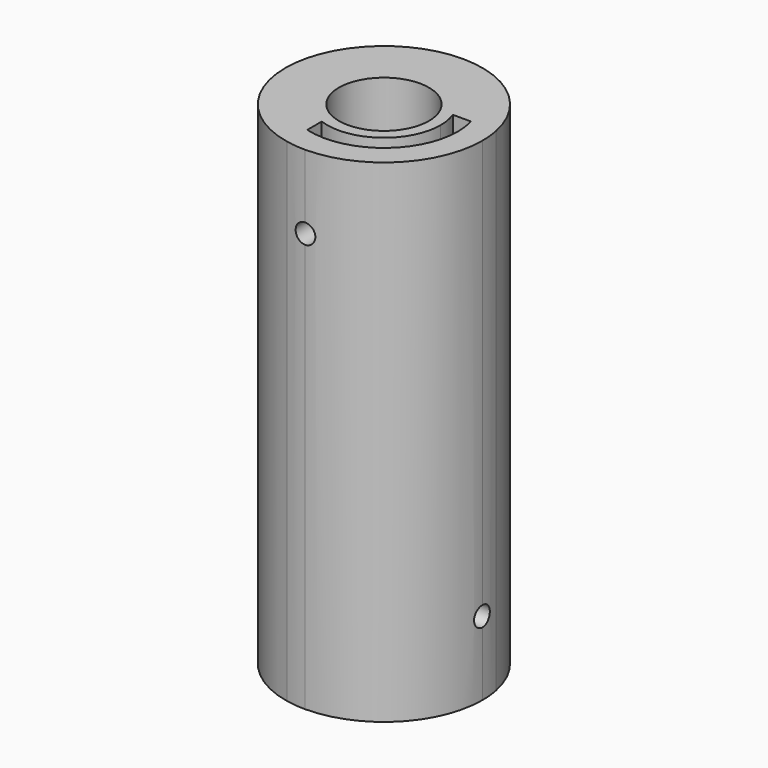
from build123d import *
from build123d import SkipClean  # not in build123d's __all__

# Parameters (mm, degrees)
F1_DEPTH = 100
F2_R     = 2
F3_DEPTH = 15
F4_R     = 2
F5_DEPTH = 6
F6_DEPTH = 100.0010001
F8_R     = 2
F9_DEPTH = 10


with BuildPart() as f1:
    # F0 (on Top) → F1 (new body)
    with BuildSketch(Plane.XY):
        with BuildLine():
            ThreePointArc((-36.113968879, 21.9828632864), (-38.5839959268, 36.6822584753), (-23.884600738, 34.2122314274))
            Line((-23.884600738, 34.2122314274), (-21.3320395526, 34.2122314274))
            ThreePointArc((-21.3320395526, 34.2122314274), (-40.2456968626, 38.3439594111), (-36.113968879, 19.430302101))
            Line((-36.113968879, 19.430302101), (-36.113968879, 21.9828632864))
        make_face()
        with BuildLine():
            ThreePointArc((-23.884600738, 34.2122314274), (-23.1970967118, 32.2645205774), (-22.963968879, 30.2122314274))
            ThreePointArc((-22.963968879, 30.2122314274), (-27.2599756775, 22.4558630762), (-36.113968879, 21.9828632864))
            Line((-36.113968879, 21.9828632864), (-36.113968879, 19.430302101))
            ThreePointArc((-36.113968879, 19.430302101), (-25.5470061107, 20.7716276332), (-20.613968879, 30.2122314274))
            ThreePointArc((-20.613968879, 30.2122314274), (-20.7949100123, 32.2442024836), (-21.3320395526, 34.2122314274))
            Line((-21.3320395526, 34.2122314274), (-23.884600738, 34.2122314274))
        make_face()
        with BuildLine():
            ThreePointArc((-52.113968879, 30.2122314274), (-46.2561045027, 44.3543670512), (-32.113968879, 50.2122314274))
            Line((-32.113968879, 50.2122314274), (-52.113968879, 50.2122314274))
            Line((-52.113968879, 50.2122314274), (-52.113968879, 30.2122314274))
        make_face()
        with BuildLine():
            ThreePointArc((-32.113968879, 50.2122314274), (-19.4648582383, 45.7041648123), (-12.5180509367, 34.2122314274))
            ThreePointArc((-12.5180509367, 34.2122314274), (-12.2152458189, 32.2224106675), (-12.113968879, 30.2122314274))
            Line((-12.113968879, 30.2122314274), (-12.113968879, 50.2122314274))
            Line((-12.113968879, 50.2122314274), (-32.113968879, 50.2122314274))
        make_face()
        with BuildLine():
            Line((-12.113968879, 10.2122314274), (-12.113968879, 30.2122314274))
            ThreePointArc((-12.113968879, 30.2122314274), (-17.9718332553, 16.0700958037), (-32.113968879, 10.2122314274))
            Line((-32.113968879, 10.2122314274), (-12.113968879, 10.2122314274))
        make_face()
        with BuildLine():
            ThreePointArc((-32.113968879, 10.2122314274), (-34.1241481191, 10.3135083673), (-36.113968879, 10.6163134852))
            ThreePointArc((-36.113968879, 10.6163134852), (-47.6059022638, 17.5631207868), (-52.113968879, 30.2122314274))
            Line((-52.113968879, 30.2122314274), (-52.113968879, 10.2122314274))
            Line((-52.113968879, 10.2122314274), (-32.113968879, 10.2122314274))
        make_face()
        with BuildLine():
            ThreePointArc((-36.113968879, 15.7553991326), (-42.7205705968, 40.8188331452), (-17.6571365842, 34.2122314274))
            Line((-17.6571365842, 34.2122314274), (-12.5180509367, 34.2122314274))
            ThreePointArc((-12.5180509367, 34.2122314274), (-19.4648582383, 45.7041648123), (-32.113968879, 50.2122314274))
            ThreePointArc((-32.113968879, 50.2122314274), (-46.2561045027, 44.3543670512), (-52.113968879, 30.2122314274))
            ThreePointArc((-52.113968879, 30.2122314274), (-47.6059022638, 17.5631207868), (-36.113968879, 10.6163134852))
            Line((-36.113968879, 10.6163134852), (-36.113968879, 15.7553991326))
        make_face()
        with BuildLine():
            Line((-12.5180509367, 34.2122314274), (-17.6571365842, 34.2122314274))
            ThreePointArc((-17.6571365842, 34.2122314274), (-17.2503810816, 32.2305866462), (-17.113968879, 30.2122314274))
            ThreePointArc((-17.113968879, 30.2122314274), (-23.0310178167, 18.2748950411), (-36.113968879, 15.7553991326))
            Line((-36.113968879, 15.7553991326), (-36.113968879, 10.6163134852))
            ThreePointArc((-36.113968879, 10.6163134852), (-34.1241481191, 10.3135083673), (-32.113968879, 10.2122314274))
            ThreePointArc((-32.113968879, 10.2122314274), (-17.9718332553, 16.0700958037), (-12.113968879, 30.2122314274))
            ThreePointArc((-12.113968879, 30.2122314274), (-12.2152458189, 32.2224106675), (-12.5180509367, 34.2122314274))
        make_face()
        with BuildLine():
            ThreePointArc((-36.113968879, 19.430302101), (-40.2456968626, 38.3439594111), (-21.3320395526, 34.2122314274))
            Line((-21.3320395526, 34.2122314274), (-17.6571365842, 34.2122314274))
            ThreePointArc((-17.6571365842, 34.2122314274), (-42.7205705968, 40.8188331452), (-36.113968879, 15.7553991326))
            Line((-36.113968879, 15.7553991326), (-36.113968879, 19.430302101))
        make_face()
    extrude(amount=F1_DEPTH)

    # F2 (on face) → F3 (cut)
    with BuildSketch(Plane.XZ.offset(-10.2122314274)):
        with Locations((-32.113968879, 85)):
            Circle(F2_R)
    extrude(amount=-F3_DEPTH, mode=Mode.SUBTRACT)

    # F4 (on face) → F5 (cut)
    with BuildSketch(Plane.YZ.offset(-12.113968879)):
        with Locations((30.2122314274, 15)):
            Circle(F4_R)
    extrude(amount=-F5_DEPTH, mode=Mode.SUBTRACT)

    # F0 (on Top) → F6 (cut, through all)
    with BuildSketch(Plane.XY):
        with BuildLine():
            Line((-12.113968879, 10.2122314274), (-12.113968879, 30.2122314274))
            ThreePointArc((-12.113968879, 30.2122314274), (-17.9718332553, 16.0700958037), (-32.113968879, 10.2122314274))
            Line((-32.113968879, 10.2122314274), (-12.113968879, 10.2122314274))
        make_face()
        with BuildLine():
            ThreePointArc((-32.113968879, 10.2122314274), (-34.1241481191, 10.3135083673), (-36.113968879, 10.6163134852))
            ThreePointArc((-36.113968879, 10.6163134852), (-47.6059022638, 17.5631207868), (-52.113968879, 30.2122314274))
            Line((-52.113968879, 30.2122314274), (-52.113968879, 10.2122314274))
            Line((-52.113968879, 10.2122314274), (-32.113968879, 10.2122314274))
        make_face()
        with BuildLine():
            ThreePointArc((-52.113968879, 30.2122314274), (-46.2561045027, 44.3543670512), (-32.113968879, 50.2122314274))
            Line((-32.113968879, 50.2122314274), (-52.113968879, 50.2122314274))
            Line((-52.113968879, 50.2122314274), (-52.113968879, 30.2122314274))
        make_face()
        with BuildLine():
            ThreePointArc((-32.113968879, 50.2122314274), (-19.4648582383, 45.7041648123), (-12.5180509367, 34.2122314274))
            ThreePointArc((-12.5180509367, 34.2122314274), (-12.2152458189, 32.2224106675), (-12.113968879, 30.2122314274))
            Line((-12.113968879, 30.2122314274), (-12.113968879, 50.2122314274))
            Line((-12.113968879, 50.2122314274), (-32.113968879, 50.2122314274))
        make_face()
    with SkipClean():  # cleaning this boolean's faces spoils the solid; the shape is the same uncleaned
        extrude(amount=F6_DEPTH, mode=Mode.SUBTRACT)

    # F8 (on offset) → F9 (cut)
    with BuildSketch(Plane.YZ.offset(-30)):
        with Locations((30.0163067877, 85.1406082511)):
            Circle(F8_R)
    with SkipClean():  # cleaning this boolean's faces spoils the solid; the shape is the same uncleaned
        extrude(amount=F9_DEPTH, mode=Mode.SUBTRACT)


solid = f1.part
